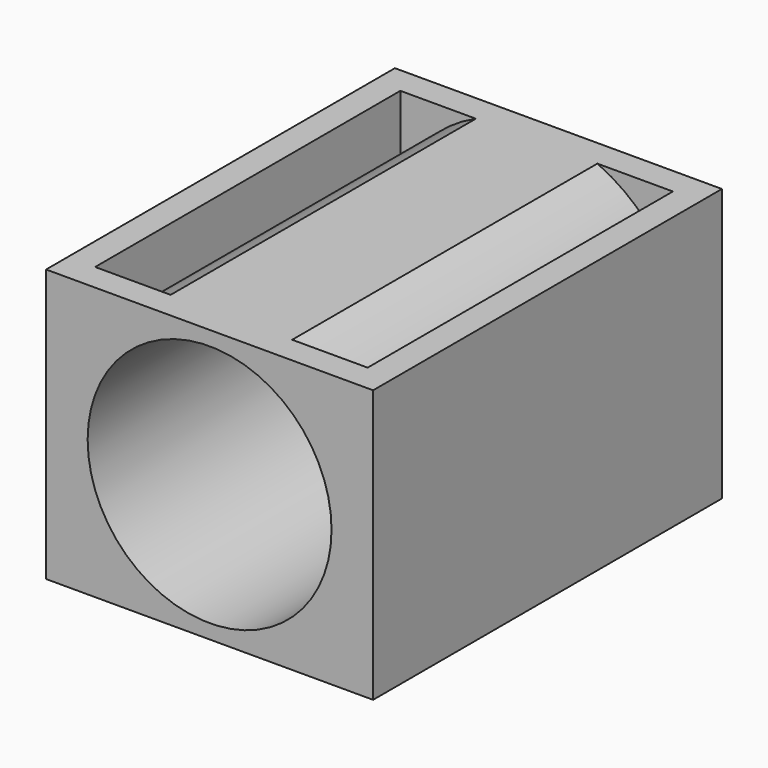
from build123d import *

# Parameters (mm, degrees)
F0_W     = 30
F0_H     = 25
F1_DEPTH = 40
F2_R     = 11.1868683522
F3_DEPTH = 37
F4_T     = 2.5


# Not quite as in the source:
# - a shell that OpenCascade refuses in one call is made with other operations: the cavity is built on its own and cut out


with BuildPart() as f1:
    # F0 (on Front) → F1 (new body)
    with BuildSketch(Plane.XZ):
        Rectangle(F0_W, F0_H)
    extrude(amount=F1_DEPTH)

    # F2 (on face) → F3 (cut)
    with BuildSketch(Plane.XZ.offset(40)):
        Circle(F2_R)
    extrude(amount=-F3_DEPTH, mode=Mode.SUBTRACT)

    # F4: shell of thickness 2.5, made by hand


with BuildPart() as f4_core1:
    # F4_t2: copy of F1
    add(f1.part)

    # the walls: a layer under each face that stays
    f4_faces = [f4_core1.faces().sort_by_distance(p)[0] for p in [
        (0, -20, -12.5),
        (-15, -20, 0),
        (15, -20, 0),
        (0, 0, 0),
        (-10, -40, -8.3333333333),
        (-11.1868683522, -21.5, 0),
        (0, -3, 0),
    ]]
    thicken(f4_faces, amount=-F4_T, mode=Mode.SUBTRACT)

    # F4_s3 → F4_t4 (revolve, cut)
    with BuildSketch(Plane.XY):
        Polygon((11.1618683522, -3.025), (13.6868683522, -3), (13.6868683522, -0.5), (11.1868683522, -0.5), align=None)
    revolve(axis=Axis((0, -3, 0), (0, -1, 0)), mode=Mode.SUBTRACT)


with BuildPart() as f1_1:
    add(f1.part)

    # what is left inside the walls is the cavity
    f4_cavity = [f4_core1.part.solids().sort_by_distance(p)[0] for p in [
        (-9.695755, -25.833333, 9.695755),
        (9.695755, -25.833333, 9.695755),
        (11.164727, -25.833333, -7.960164),
        (-11.164727, -25.833333, -7.960164),
    ]]
    add(f4_cavity, mode=Mode.SUBTRACT)


solid = f1_1.part
